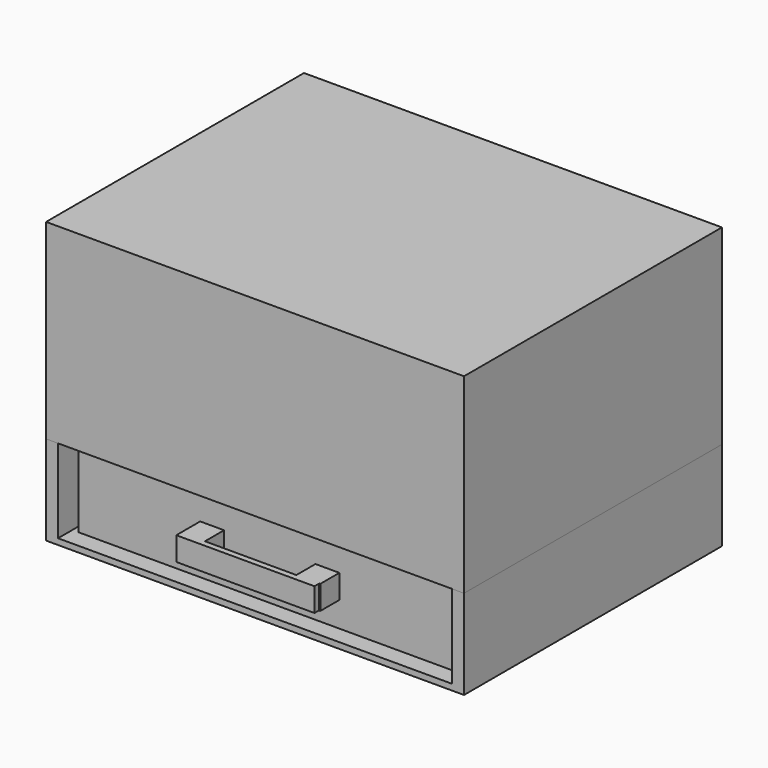
from build123d import *

# Parameters (mm, degrees)
F0_W      = 406.4
F0_H      = 304.8
F1_DEPTH  = 6.35
F2_W      = 12.4951104045
F2_H      = 279.4
F2_W_2    = 13.0043203354
F3_DEPTH  = 76.2
F4_W      = 444.5
F4_H      = 342.9
F5_DEPTH  = 6.35
F6_W      = 419.1
F6_H      = 11.9031353712
F7_DEPTH  = 88.9
F8_W      = 444.5
F8_H      = 342.9
F9_DEPTH  = 203.2
F10_W     = 25.4
F10_H     = 25.4
F11_DEPTH = 25.4
F12_W     = 146.9787295926
F12_H     = 25.0639826562
F13_DEPTH = 6.35


# Not quite as in the source:
# - a length typed as a fraction of an inch, garbled in the dataset ("3 / 203.2 mm" for 3/8 in), is restored


with BuildPart() as f1:
    # F0 (on Top) → F1 (new body)
    with BuildSketch(Plane.XY):
        Rectangle(F0_W, F0_H)
    extrude(amount=F1_DEPTH)

    # F2 (on face) → F3 (join)
    with BuildSketch(Plane.XY.offset(6.35)):
        Polygon((-203.2, -139.7), (-203.2, -152.4), (203.2, -152.4), (203.2, -139.7), (190.1956796646, -139.7), (-190.7048895955, -139.7), align=None)
        with Locations((-196.9524447978, 0)):
            Rectangle(F2_W, F2_H)
        with Locations((196.6978398323, 0)):
            Rectangle(F2_W_2, F2_H)
        Polygon((-203.2, 152.4), (-203.2, 139.7), (-190.7048895955, 139.7), (190.1956796646, 139.7), (203.2, 139.7), (203.2, 152.4), align=None)
    extrude(amount=F3_DEPTH)

    # F10 (on face) → F11 (join)
    with BuildSketch(Plane.XZ.offset(152.4)):
        with Locations((-60.9074905861, 39.5232320662)):
            Rectangle(F10_W, F10_H)
        with Locations((61.7435536951, 39.5232320662)):
            Rectangle(F10_W, F10_H)
    extrude(amount=F11_DEPTH)

    # F12 (on face) → F13 (join)
    with BuildSketch(Plane.XZ.offset(177.8)):
        with Locations((-0.1181257898, 39.6912407381)):
            Rectangle(F12_W, F12_H)
    extrude(amount=F13_DEPTH)


with BuildPart() as f5:
    # F4 (on face) → F5 (new body)
    with BuildSketch(Plane(origin=(0, 0, 0), x_dir=(1, 0, 0), z_dir=(0, 0, -1))):
        Rectangle(F4_W, F4_H)
    extrude(amount=F5_DEPTH)

    # F6 (on face) → F7 (join)
    with BuildSketch(Plane.XY):
        Polygon((209.55, -171.45), (222.25, -171.45), (222.25, 171.45), (209.55, 171.45), (209.55, 159.5468646288), (209.55, -158.75), align=None)
        with Locations((0, 165.4984323144)):
            Rectangle(F6_W, F6_H)
        Polygon((-209.55, 159.5468646288), (-209.55, 171.45), (-222.25, 171.45), (-222.25, -171.45), (-209.55, -171.45), align=None)
    extrude(amount=F7_DEPTH)


with BuildPart() as f9:
    # F8 (on face) → F9 (new body)
    with BuildSketch(Plane.XY.offset(88.9)):
        Rectangle(F8_W, F8_H)
    extrude(amount=F9_DEPTH)


solid = Compound([f1.part, f5.part, f9.part])
